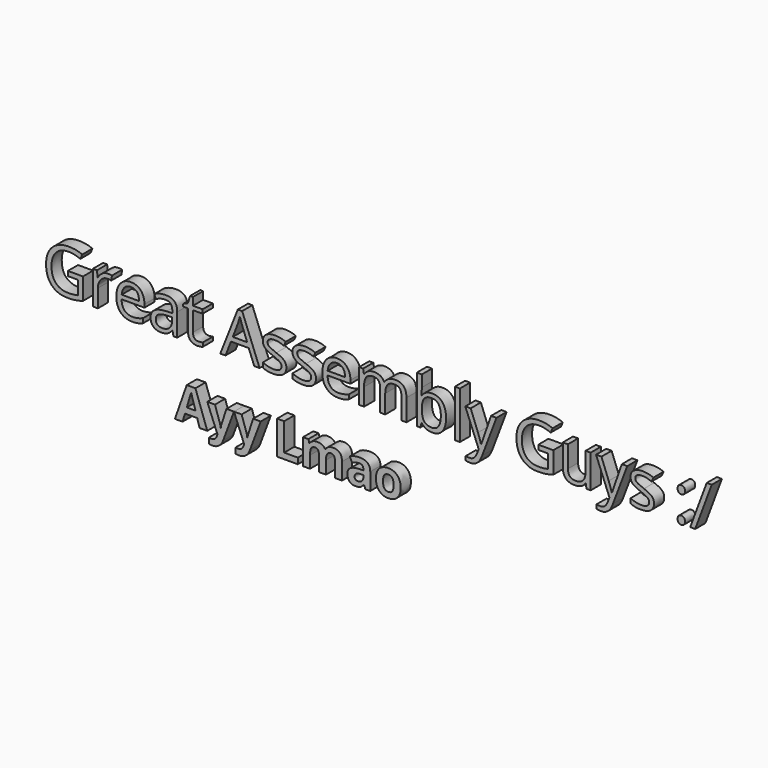
from build123d import *

# Parameters (mm, degrees)
F0_TEXT_SIZE = 123.805440833
F1_DEPTH     = 25.4
F2_TEXT_SIZE = 93.5354994403
F3_DEPTH     = 25.4


# Not quite as in the source:
# - Text() gives the source's letters only with a copy of the font that has no kerning and outlines rounded to 1/6400 em; it was checked with that copy


with BuildPart() as f1:
    # F0 (on Front) → F1 (new body)
    with BuildSketch(Plane.XZ):
        with Locations((-525.9469747543, -82.4935734272)):
            Text('Great Assembly Guys :/', F0_TEXT_SIZE, font='Open Sans', text_align=(TextAlign.LEFT, TextAlign.BOTTOM))
    extrude(amount=F1_DEPTH)


with BuildPart() as f3:
    # F2 (on Front) → F3 (new body)
    with BuildSketch(Plane.XZ):
        with Locations((-261.548101902, -226.5308946371)):
            Text('Ayy Lmao', F2_TEXT_SIZE, font='Open Sans', font_style=FontStyle.BOLD, text_align=(TextAlign.LEFT, TextAlign.BOTTOM))
    extrude(amount=F3_DEPTH)


solid = Compound([f1.part, f3.part])
